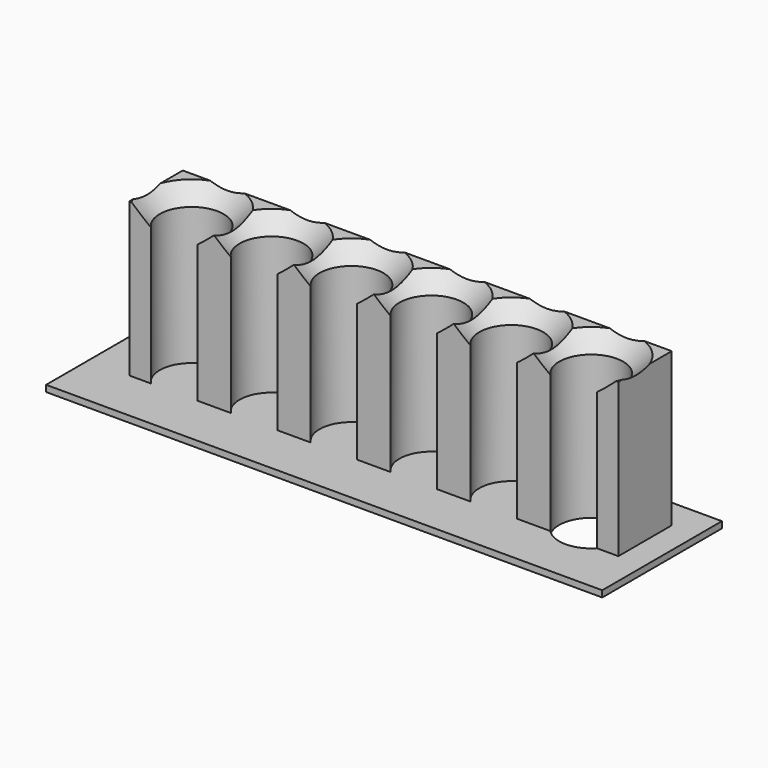
from build123d import *

# Parameters (mm, degrees)
F1_DEPTH     = 50
F0_W         = 174.0209832788
F0_H         = 46.8094409443
F2_DEPTH     = 2
F3_T2_ANGLE  = 297.2148412711
F3_T4_ANGLE  = 297.2148412711
F3_T6_ANGLE  = 297.2148412711
F3_T8_ANGLE  = 297.2148412711
F3_T10_ANGLE = 297.2148412711
F3_T12_ANGLE = 297.2148412711
F3_T14_ANGLE = 117.0391625113
F3_T16_ANGLE = 117.0391625113
F3_T18_ANGLE = 117.0391625113
F3_T20_ANGLE = 117.0391625113
F3_T22_ANGLE = 117.0391625113
F3_T24_ANGLE = 117.0391625113


# Not quite as in the source:
# - a fillet or chamfer that OpenCascade refuses, or shapes differently, is made with other operations: its cross-section is extruded or revolved along the edge and cut away or added


with BuildPart() as f1:
    # F0 (on Top) → F1 (new body)
    with BuildSketch(Plane.XY):
        with BuildLine():
            ThreePointArc((-63.3511276029, 24.1111628711), (-59.7746098829, 40.2694854105), (-46.0804665685, 30.9768375009))
            ThreePointArc((-46.0804665685, 30.9768375009), (-46.7878186589, 27.2826941865), (-48.809805534, 24.1111628711))
            Line((-48.809805534, 24.1111628711), (-38.3511276029, 24.1111628711))
            ThreePointArc((-38.3511276029, 24.1111628711), (-34.7746098829, 40.2694854105), (-21.0804665685, 30.9768375009))
            ThreePointArc((-21.0804665685, 30.9768375009), (-21.7878186589, 27.2826941865), (-23.809805534, 24.1111628711))
            Line((-23.809805534, 24.1111628711), (-13.3511276029, 24.1111628711))
            ThreePointArc((-13.3511276029, 24.1111628711), (-9.7746098829, 40.2694854105), (3.9195334315, 30.9768375009))
            ThreePointArc((3.9195334315, 30.9768375009), (3.2121813411, 27.2826941865), (1.190194466, 24.1111628711))
            Line((1.190194466, 24.1111628711), (11.6488723971, 24.1111628711))
            ThreePointArc((11.6488723971, 24.1111628711), (15.2253901171, 40.2694854105), (28.9195334315, 30.9768375009))
            ThreePointArc((28.9195334315, 30.9768375009), (28.2121813411, 27.2826941865), (26.190194466, 24.1111628711))
            Line((26.190194466, 24.1111628711), (36.6488723971, 24.1111628711))
            ThreePointArc((36.6488723971, 24.1111628711), (40.2253901171, 40.2694854105), (53.9195334315, 30.9768375009))
            ThreePointArc((53.9195334315, 30.9768375009), (53.2121813411, 27.2826941865), (51.190194466, 24.1111628711))
            Line((51.190194466, 24.1111628711), (61.6488723971, 24.1111628711))
            ThreePointArc((61.6488723971, 24.1111628711), (65.2253901171, 40.2694854105), (78.9195334315, 30.9768375009))
            ThreePointArc((78.9195334315, 30.9768375009), (78.2121813411, 27.2826941865), (76.190194466, 24.1111628711))
            Line((76.190194466, 24.1111628711), (82.9195334315, 24.1111628711))
            Line((82.9195334315, 24.1111628711), (82.9195334315, 44.9768375009))
            Line((82.9195334315, 44.9768375009), (-70.0804665685, 44.9768375009))
            Line((-70.0804665685, 44.9768375009), (-70.0804665685, 24.1111628711))
            Line((-70.0804665685, 24.1111628711), (-63.3511276029, 24.1111628711))
        make_face()
    extrude(amount=F1_DEPTH)

    # F0 (on Top) → F2 (join)
    with BuildSketch(Plane.XY):
        with Locations((4.097443074, 30.9768363368)):
            Rectangle(F0_W, F0_H)
        Polygon((-70.0804665685, 16.9768375009), (-70.0804665685, 24.1111628711), (-70.0804665685, 44.9768375009), (82.9195334315, 44.9768375009), (82.9195334315, 24.1111628711), (82.9195334315, 16.9768375009), align=None, mode=Mode.SUBTRACT)
        with BuildLine():
            ThreePointArc((-48.809805534, 24.1111628711), (-56.0804665685, 20.9768375009), (-63.3511276029, 24.1111628711))
            Line((-63.3511276029, 24.1111628711), (-70.0804665685, 24.1111628711))
            Line((-70.0804665685, 24.1111628711), (-70.0804665685, 16.9768375009))
            Line((-70.0804665685, 16.9768375009), (82.9195334315, 16.9768375009))
            Line((82.9195334315, 16.9768375009), (82.9195334315, 24.1111628711))
            Line((82.9195334315, 24.1111628711), (76.190194466, 24.1111628711))
            ThreePointArc((76.190194466, 24.1111628711), (68.9195334315, 20.9768375009), (61.6488723971, 24.1111628711))
            Line((61.6488723971, 24.1111628711), (51.190194466, 24.1111628711))
            ThreePointArc((51.190194466, 24.1111628711), (43.9195334315, 20.9768375009), (36.6488723971, 24.1111628711))
            Line((36.6488723971, 24.1111628711), (26.190194466, 24.1111628711))
            ThreePointArc((26.190194466, 24.1111628711), (18.9195334315, 20.9768375009), (11.6488723971, 24.1111628711))
            Line((11.6488723971, 24.1111628711), (1.190194466, 24.1111628711))
            ThreePointArc((1.190194466, 24.1111628711), (-6.0804665685, 20.9768375009), (-13.3511276029, 24.1111628711))
            Line((-13.3511276029, 24.1111628711), (-23.809805534, 24.1111628711))
            ThreePointArc((-23.809805534, 24.1111628711), (-31.0804665685, 20.9768375009), (-38.3511276029, 24.1111628711))
            Line((-38.3511276029, 24.1111628711), (-48.809805534, 24.1111628711))
        make_face()
        with BuildLine():
            ThreePointArc((-48.809805534, 24.1111628711), (-46.7878186589, 27.2826941865), (-46.0804665685, 30.9768375009))
            ThreePointArc((-46.0804665685, 30.9768375009), (-59.7746098829, 40.2694854105), (-63.3511276029, 24.1111628711))
            Line((-63.3511276029, 24.1111628711), (-48.809805534, 24.1111628711))
        make_face()
        with BuildLine():
            Line((-48.809805534, 24.1111628711), (-63.3511276029, 24.1111628711))
            ThreePointArc((-63.3511276029, 24.1111628711), (-56.0804665685, 20.9768375009), (-48.809805534, 24.1111628711))
        make_face()
        with BuildLine():
            ThreePointArc((-21.0804665685, 30.9768375009), (-34.7746098829, 40.2694854105), (-38.3511276029, 24.1111628711))
            Line((-38.3511276029, 24.1111628711), (-23.809805534, 24.1111628711))
            ThreePointArc((-23.809805534, 24.1111628711), (-21.7878186589, 27.2826941865), (-21.0804665685, 30.9768375009))
        make_face()
        with BuildLine():
            Line((-23.809805534, 24.1111628711), (-38.3511276029, 24.1111628711))
            ThreePointArc((-38.3511276029, 24.1111628711), (-31.0804665685, 20.9768375009), (-23.809805534, 24.1111628711))
        make_face()
        with BuildLine():
            ThreePointArc((3.9195334315, 30.9768375009), (-9.7746098829, 40.2694854105), (-13.3511276029, 24.1111628711))
            Line((-13.3511276029, 24.1111628711), (1.190194466, 24.1111628711))
            ThreePointArc((1.190194466, 24.1111628711), (3.2121813411, 27.2826941865), (3.9195334315, 30.9768375009))
        make_face()
        with BuildLine():
            Line((1.190194466, 24.1111628711), (-13.3511276029, 24.1111628711))
            ThreePointArc((-13.3511276029, 24.1111628711), (-6.0804665685, 20.9768375009), (1.190194466, 24.1111628711))
        make_face()
        with BuildLine():
            ThreePointArc((28.9195334315, 30.9768375009), (15.2253901171, 40.2694854105), (11.6488723971, 24.1111628711))
            Line((11.6488723971, 24.1111628711), (26.190194466, 24.1111628711))
            ThreePointArc((26.190194466, 24.1111628711), (28.2121813411, 27.2826941865), (28.9195334315, 30.9768375009))
        make_face()
        with BuildLine():
            Line((26.190194466, 24.1111628711), (11.6488723971, 24.1111628711))
            ThreePointArc((11.6488723971, 24.1111628711), (18.9195334315, 20.9768375009), (26.190194466, 24.1111628711))
        make_face()
        with BuildLine():
            Line((36.6488723971, 24.1111628711), (51.190194466, 24.1111628711))
            ThreePointArc((51.190194466, 24.1111628711), (53.2121813411, 27.2826941865), (53.9195334315, 30.9768375009))
            ThreePointArc((53.9195334315, 30.9768375009), (40.2253901171, 40.2694854105), (36.6488723971, 24.1111628711))
        make_face()
        with BuildLine():
            ThreePointArc((36.6488723971, 24.1111628711), (43.9195334315, 20.9768375009), (51.190194466, 24.1111628711))
            Line((51.190194466, 24.1111628711), (36.6488723971, 24.1111628711))
        make_face()
    extrude(amount=F2_DEPTH)

    # F3: chamfer of 5 on 6 edges, made by hand

    # F3_s1 → F3_t2 (revolve, cut)
    with BuildSketch(Plane(origin=(-31.7529692139, -16.3292082814, 0), x_dir=(0, 0, 1), z_dir=(0.8892979418, 0.4573282964, 0))):
        Polygon((45, -43.1948220704), (50, -38.1948220704), (50, -43.1948220704), align=None)
    revolve(axis=Axis((-56.0804665685, 30.9768375009, 50), (0, 0, -1)), revolution_arc=F3_T2_ANGLE, mode=Mode.SUBTRACT)

    # F3_s3 → F3_t4 (revolve, cut)
    with BuildSketch(Plane(origin=(-11.981698481, -6.1616804635, 0), x_dir=(0, 0, 1), z_dir=(0.8892979418, 0.4573282964, 0))):
        Polygon((45, -31.7616146605), (50, -26.7616146605), (50, -31.7616146605), align=None)
    revolve(axis=Axis((-31.0804665685, 30.9768375009, 50), (0, 0, -1)), revolution_arc=F3_T4_ANGLE, mode=Mode.SUBTRACT)

    # F3_s5 → F3_t6 (revolve, cut)
    with BuildSketch(Plane(origin=(7.7895722518, 4.0058473545, 0), x_dir=(0, 0, 1), z_dir=(0.8892979418, 0.4573282964, 0))):
        Polygon((45, -20.3284072505), (50, -15.3284072505), (50, -20.3284072505), align=None)
    revolve(axis=Axis((-6.0804665685, 30.9768375009, 50), (0, 0, -1)), revolution_arc=F3_T6_ANGLE, mode=Mode.SUBTRACT)

    # F3_s7 → F3_t8 (revolve, cut)
    with BuildSketch(Plane(origin=(27.5608429847, 14.1733751725, 0), x_dir=(0, 0, 1), z_dir=(0.8892979418, 0.4573282964, 0))):
        Polygon((45, -8.8951998406), (50, -3.8951998406), (50, -8.8951998406), align=None)
    revolve(axis=Axis((18.9195334315, 30.9768375009, 50), (0, 0, -1)), revolution_arc=F3_T8_ANGLE, mode=Mode.SUBTRACT)

    # F3_s9 → F3_t10 (revolve, cut)
    with BuildSketch(Plane(origin=(47.3321137176, 24.3409029904, 0), x_dir=(0, 0, 1), z_dir=(0.8892979418, 0.4573282964, 0))):
        Polygon((45, 2.5380075693), (50, 7.5380075693), (50, 2.5380075693), align=None)
    revolve(axis=Axis((43.9195334315, 30.9768375009, 50), (0, 0, -1)), revolution_arc=F3_T10_ANGLE, mode=Mode.SUBTRACT)

    # F3_s11 → F3_t12 (revolve, cut)
    with BuildSketch(Plane(origin=(67.1033844505, 34.5084308084, 0), x_dir=(0, 0, 1), z_dir=(0.8892979418, 0.4573282964, 0))):
        Polygon((45, 13.9712149792), (50, 18.9712149792), (50, 13.9712149792), align=None)
    revolve(axis=Axis((68.9195334315, 30.9768375009, 50), (0, 0, -1)), revolution_arc=F3_T12_ANGLE, mode=Mode.SUBTRACT)

    # F3_s13 → F3_t14 (revolve, cut)
    with BuildSketch(Plane.XZ.offset(-30.9768375009)):
        Polygon((78.9195334315, 45), (83.9195334315, 50), (78.9195334315, 50), align=None)
    revolve(axis=Axis((68.9195334315, 30.9768375009, 50), (0, 0, -1)), revolution_arc=F3_T14_ANGLE, mode=Mode.SUBTRACT)

    # F3_s15 → F3_t16 (revolve, cut)
    with BuildSketch(Plane.XZ.offset(-30.9768375009)):
        Polygon((53.9195334315, 45), (58.9195334315, 50), (53.9195334315, 50), align=None)
    revolve(axis=Axis((43.9195334315, 30.9768375009, 50), (0, 0, -1)), revolution_arc=F3_T16_ANGLE, mode=Mode.SUBTRACT)

    # F3_s17 → F3_t18 (revolve, cut)
    with BuildSketch(Plane.XZ.offset(-30.9768375009)):
        Polygon((28.9195334315, 45), (33.9195334315, 50), (28.9195334315, 50), align=None)
    revolve(axis=Axis((18.9195334315, 30.9768375009, 50), (0, 0, -1)), revolution_arc=F3_T18_ANGLE, mode=Mode.SUBTRACT)

    # F3_s19 → F3_t20 (revolve, cut)
    with BuildSketch(Plane.XZ.offset(-30.9768375009)):
        Polygon((3.9195334315, 45), (8.9195334315, 50), (3.9195334315, 50), align=None)
    revolve(axis=Axis((-6.0804665685, 30.9768375009, 50), (0, 0, -1)), revolution_arc=F3_T20_ANGLE, mode=Mode.SUBTRACT)

    # F3_s21 → F3_t22 (revolve, cut)
    with BuildSketch(Plane.XZ.offset(-30.9768375009)):
        Polygon((-21.0804665685, 45), (-16.0804665685, 50), (-21.0804665685, 50), align=None)
    revolve(axis=Axis((-31.0804665685, 30.9768375009, 50), (0, 0, -1)), revolution_arc=F3_T22_ANGLE, mode=Mode.SUBTRACT)

    # F3_s23 → F3_t24 (revolve, cut)
    with BuildSketch(Plane.XZ.offset(-30.9768375009)):
        Polygon((-46.0804665685, 45), (-41.0804665685, 50), (-46.0804665685, 50), align=None)
    revolve(axis=Axis((-56.0804665685, 30.9768375009, 50), (0, 0, -1)), revolution_arc=F3_T24_ANGLE, mode=Mode.SUBTRACT)


solid = f1.part
